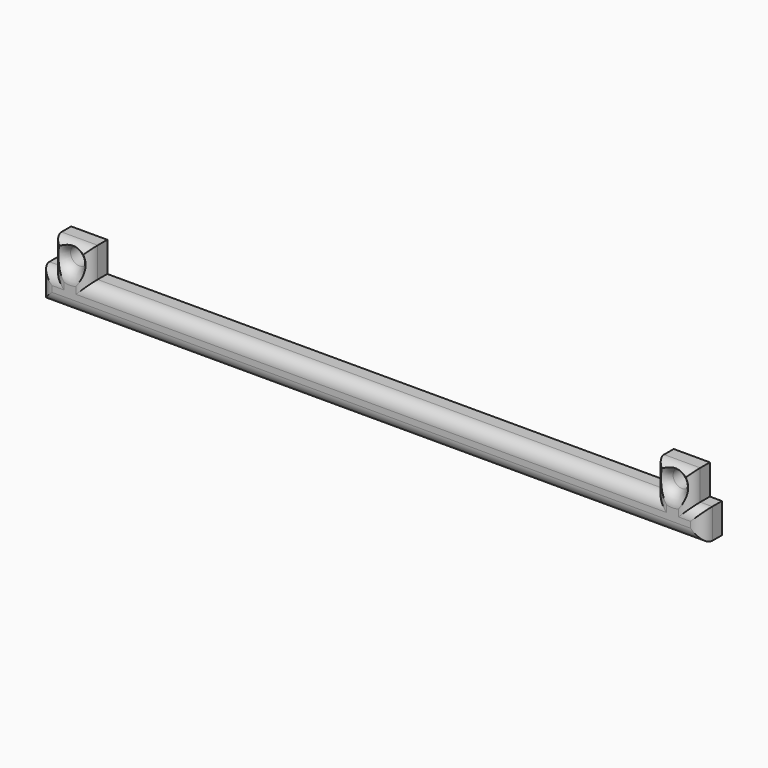
from build123d import *

# Parameters (mm, degrees)
F0_R         = 1.5
F1_DEPTH     = 4
F2_T1_DEPTH  = 15
F2_T3_DEPTH  = 120
F2_T5_DEPTH  = 7
F2_T7_DEPTH  = 10
F2_T9_DEPTH  = 16
F2_T11_DEPTH = 94
F2_T13_DEPTH = 16
F2_T15_DEPTH = 7
F2_T25_DEPTH = 12
F2_T29_DEPTH = 15
F2_T36_DEPTH = 15
F2_T40_DEPTH = 99
F2_T47_DEPTH = 99
F2_T51_DEPTH = 15
F2_T58_DEPTH = 15
F2_T62_DEPTH = 12


# Not quite as in the source:
# - a fillet or chamfer that OpenCascade refuses, or shapes differently, is made with other operations: its cross-section is extruded or revolved along the edge and cut away or added


with BuildPart() as f1:
    # F0 (on Front) → F1 (new body)
    with BuildSketch(Plane.XZ):
        Polygon((-55, 5), (-55, 0), (55, 0), (55, 5), (53, 5), (53, 10), (47, 10), (47, 5), (-47, 5), (-47, 10), (-53, 10), (-53, 5), align=None)
        with Locations((-50, 7.5)):
            Circle(F0_R, mode=Mode.SUBTRACT)
        with Locations((50, 7.5)):
            Circle(F0_R, mode=Mode.SUBTRACT)
    extrude(amount=F1_DEPTH)

    # F2: fillet of radius 2 on 14 edges, made by hand

    # F2_s2 → F2_t1 (cut)
    with BuildSketch(Plane.XY.offset(-5)):
        with BuildLine():
            ThreePointArc((-55, -2), (-54.4142135624, -3.4142135624), (-53, -4))
            Line((-53, -4), (-55, -4))
            Line((-55, -4), (-55, -2))
        make_face()
        with BuildLine():
            ThreePointArc((55, -2), (54.4142135624, -3.4142135624), (53, -4))
            Line((53, -4), (55, -4))
            Line((55, -4), (55, -2))
        make_face()
    extrude(amount=F2_T1_DEPTH, mode=Mode.SUBTRACT)

    # F2_s4 → F2_t3 (cut)
    with BuildSketch(Plane.YZ.offset(-60)):
        with BuildLine():
            ThreePointArc((-2, 0), (-3.4142135624, 0.5857864376), (-4, 2))
            Line((-4, 2), (-4, 0))
            Line((-4, 0), (-2, 0))
        make_face()
    extrude(amount=F2_T3_DEPTH, mode=Mode.SUBTRACT)

    # F2_s6 → F2_t5 (cut)
    with BuildSketch(Plane.YZ.offset(53)):
        with BuildLine():
            ThreePointArc((-2, 5), (-3.4142135624, 4.4142135624), (-4, 3))
            Line((-4, 3), (-4, 5))
            Line((-4, 5), (-2, 5))
        make_face()
    extrude(amount=F2_T5_DEPTH, mode=Mode.SUBTRACT)

    # F2_s8 → F2_t7 (cut)
    with BuildSketch(Plane.XY.offset(5)):
        with BuildLine():
            ThreePointArc((53, -2), (52.4142135624, -3.4142135624), (51, -4))
            Line((51, -4), (53, -4))
            Line((53, -4), (53, -2))
        make_face()
        with BuildLine():
            ThreePointArc((47, -2), (47.5857864376, -3.4142135624), (49, -4))
            Line((49, -4), (47, -4))
            Line((47, -4), (47, -2))
        make_face()
        with BuildLine():
            ThreePointArc((-47, -2), (-47.5857864376, -3.4142135624), (-49, -4))
            Line((-49, -4), (-47, -4))
            Line((-47, -4), (-47, -2))
        make_face()
        with BuildLine():
            ThreePointArc((-53, -2), (-52.4142135624, -3.4142135624), (-51, -4))
            Line((-51, -4), (-53, -4))
            Line((-53, -4), (-53, -2))
        make_face()
    extrude(amount=F2_T7_DEPTH, mode=Mode.SUBTRACT)

    # F2_s10 → F2_t9 (cut)
    with BuildSketch(Plane.YZ.offset(42)):
        with BuildLine():
            ThreePointArc((-2, 10), (-3.4142135624, 9.4142135624), (-4, 8))
            Line((-4, 8), (-4, 10))
            Line((-4, 10), (-2, 10))
        make_face()
    extrude(amount=F2_T9_DEPTH, mode=Mode.SUBTRACT)

    # F2_s12 → F2_t11 (cut)
    with BuildSketch(Plane.YZ.offset(-47)):
        with BuildLine():
            ThreePointArc((-2, 5), (-3.4142135624, 4.4142135624), (-4, 3))
            Line((-4, 3), (-4, 5))
            Line((-4, 5), (-2, 5))
        make_face()
    extrude(amount=F2_T11_DEPTH, mode=Mode.SUBTRACT)

    # F2_s14 → F2_t13 (cut)
    with BuildSketch(Plane.YZ.offset(-58)):
        with BuildLine():
            ThreePointArc((-2, 10), (-3.4142135624, 9.4142135624), (-4, 8))
            Line((-4, 8), (-4, 10))
            Line((-4, 10), (-2, 10))
        make_face()
    extrude(amount=F2_T13_DEPTH, mode=Mode.SUBTRACT)

    # F2_s16 → F2_t15 (cut)
    with BuildSketch(Plane.YZ.offset(-60)):
        with BuildLine():
            ThreePointArc((-2, 5), (-3.4142135624, 4.4142135624), (-4, 3))
            Line((-4, 3), (-4, 5))
            Line((-4, 5), (-2, 5))
        make_face()
    extrude(amount=F2_T15_DEPTH, mode=Mode.SUBTRACT)

    # F2_s17 → F2_t18 (revolve, cut)
    with BuildSketch(Plane.XY.offset(7.5)):
        with BuildLine():
            ThreePointArc((-48.5, -2), (-47.9142135624, -3.4142135624), (-46.5, -4))
            Line((-46.5, -4), (-48.5, -4))
            Line((-48.5, -4), (-48.5, -2))
        make_face()
    revolve(axis=Axis((-50, -4, 7.5), (0, -1, 0)), mode=Mode.SUBTRACT)

    # F2_s19 → F2_t20 (revolve, cut)
    with BuildSketch(Plane.XY.offset(7.5)):
        with BuildLine():
            ThreePointArc((51.5, -2), (52.0857864376, -3.4142135624), (53.5, -4))
            Line((53.5, -4), (51.5, -4))
            Line((51.5, -4), (51.5, -2))
        make_face()
    revolve(axis=Axis((50, -4, 7.5), (0, -1, 0)), mode=Mode.SUBTRACT)


with BuildPart() as f2_tool23:
    # F2_s24 → F2_t25 (new body)
    with BuildSketch(Plane.YZ.offset(60)):
        with BuildLine():
            ThreePointArc((-2, 5), (-3.4142135624, 4.4142135624), (-4, 3))
            Line((-4, 3), (-4, 5))
            Line((-4, 5), (-2, 5))
        make_face()
    extrude(amount=-F2_T25_DEPTH)

    split(bisect_by=Plane.YZ.offset(53), keep=Keep.BOTTOM)


with BuildPart() as f2_tool27:
    # F2_s28 → F2_t29 (new body)
    with BuildSketch(Plane.XY):
        with BuildLine():
            ThreePointArc((53, -2), (52.4142135624, -3.4142135624), (51, -4))
            Line((51, -4), (53, -4))
            Line((53, -4), (53, -2))
        make_face()
    extrude(amount=F2_T29_DEPTH)

    split(bisect_by=Plane.XY.offset(5), keep=Keep.BOTTOM)


with BuildPart() as f2_tool23_1:
    add(f2_tool23.part)

    # F2_t31: intersect F2_tool27
    add(f2_tool27.part, mode=Mode.INTERSECT)


with BuildPart() as f1_1:
    add(f1.part)

    # F2_t21: cut F2_tool23
    add(f2_tool23_1.part, mode=Mode.SUBTRACT)


with BuildPart() as f2_tool34:
    # F2_s35 → F2_t36 (new body)
    with BuildSketch(Plane.XY.offset(15)):
        with BuildLine():
            ThreePointArc((47, -2), (47.5857864376, -3.4142135624), (49, -4))
            Line((49, -4), (47, -4))
            Line((47, -4), (47, -2))
        make_face()
    extrude(amount=-F2_T36_DEPTH)

    split(bisect_by=Plane.XY.offset(5), keep=Keep.BOTTOM)


with BuildPart() as f2_tool38:
    # F2_s39 → F2_t40 (new body)
    with BuildSketch(Plane.YZ.offset(52)):
        with BuildLine():
            ThreePointArc((-2, 5), (-3.4142135624, 4.4142135624), (-4, 3))
            Line((-4, 3), (-4, 5))
            Line((-4, 5), (-2, 5))
        make_face()
    extrude(amount=-F2_T40_DEPTH)

    split(bisect_by=Plane.YZ.offset(47), keep=Keep.TOP)


with BuildPart() as f2_tool34_1:
    add(f2_tool34.part)

    # F2_t42: intersect F2_tool38
    add(f2_tool38.part, mode=Mode.INTERSECT)


with BuildPart() as f1_2:
    add(f1_1.part)

    # F2_t32: cut F2_tool34
    add(f2_tool34_1.part, mode=Mode.SUBTRACT)


with BuildPart() as f2_tool45:
    # F2_s46 → F2_t47 (new body)
    with BuildSketch(Plane.YZ.offset(47)):
        with BuildLine():
            ThreePointArc((-2, 5), (-3.4142135624, 4.4142135624), (-4, 3))
            Line((-4, 3), (-4, 5))
            Line((-4, 5), (-2, 5))
        make_face()
    extrude(amount=-F2_T47_DEPTH)

    split(bisect_by=Plane.YZ.offset(-47), keep=Keep.BOTTOM)


with BuildPart() as f2_tool49:
    # F2_s50 → F2_t51 (new body)
    with BuildSketch(Plane.XY):
        with BuildLine():
            ThreePointArc((-47, -2), (-47.5857864376, -3.4142135624), (-49, -4))
            Line((-49, -4), (-47, -4))
            Line((-47, -4), (-47, -2))
        make_face()
    extrude(amount=F2_T51_DEPTH)

    split(bisect_by=Plane.XY.offset(5), keep=Keep.BOTTOM)


with BuildPart() as f2_tool45_1:
    add(f2_tool45.part)

    # F2_t53: intersect F2_tool49
    add(f2_tool49.part, mode=Mode.INTERSECT)


with BuildPart() as f1_3:
    add(f1_2.part)

    # F2_t43: cut F2_tool45
    add(f2_tool45_1.part, mode=Mode.SUBTRACT)


with BuildPart() as f2_tool56:
    # F2_s57 → F2_t58 (new body)
    with BuildSketch(Plane.XY.offset(15)):
        with BuildLine():
            ThreePointArc((-53, -2), (-52.4142135624, -3.4142135624), (-51, -4))
            Line((-51, -4), (-53, -4))
            Line((-53, -4), (-53, -2))
        make_face()
    extrude(amount=-F2_T58_DEPTH)

    split(bisect_by=Plane.XY.offset(5), keep=Keep.BOTTOM)


with BuildPart() as f2_tool60:
    # F2_s61 → F2_t62 (new body)
    with BuildSketch(Plane.YZ.offset(-48)):
        with BuildLine():
            ThreePointArc((-2, 5), (-3.4142135624, 4.4142135624), (-4, 3))
            Line((-4, 3), (-4, 5))
            Line((-4, 5), (-2, 5))
        make_face()
    extrude(amount=-F2_T62_DEPTH)

    split(bisect_by=Plane.YZ.offset(-53), keep=Keep.TOP)


with BuildPart() as f2_tool56_1:
    add(f2_tool56.part)

    # F2_t64: intersect F2_tool60
    add(f2_tool60.part, mode=Mode.INTERSECT)


with BuildPart() as f1_4:
    add(f1_3.part)

    # F2_t54: cut F2_tool56
    add(f2_tool56_1.part, mode=Mode.SUBTRACT)


solid = f1_4.part
